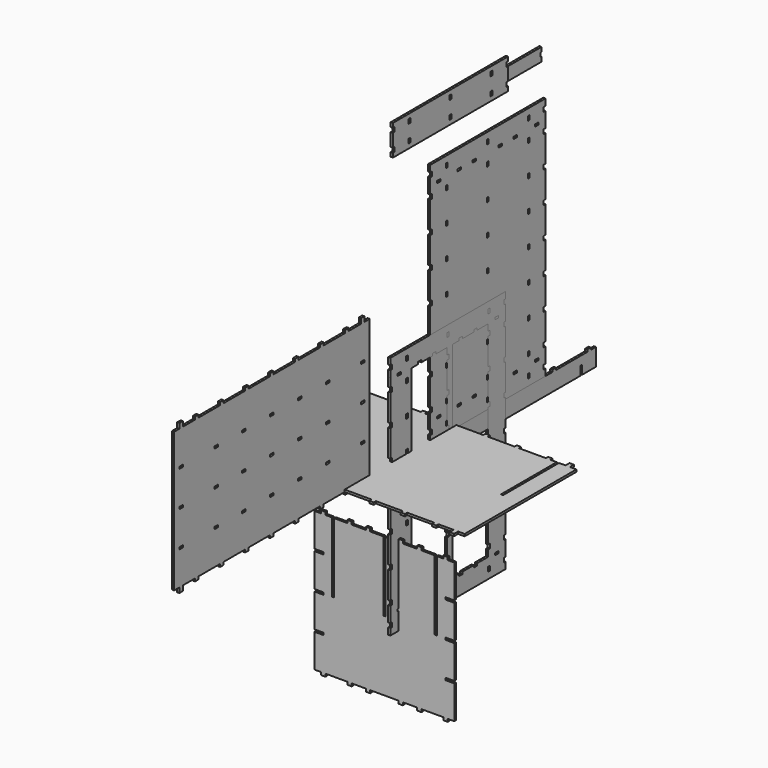
from build123d import *

# Parameters (mm, degrees)
F1_DEPTH  = 3.175
F3_DEPTH  = 3.175
F5_DEPTH  = 3.175
F6_W      = 6.35
F6_H      = 3.175
F7_DEPTH  = 3.175
F8_W      = 6.35
F8_H      = 3.175
F8_W_2    = 3.175
F8_H_2    = 6.35
F9_DEPTH  = 3.175
F10_W     = 6.35
F10_H     = 3.175
F10_W_2   = 3.175
F10_H_2   = 6.35
F11_DEPTH = 3.175
F12_W     = 3.175
F12_H     = 6.35
F13_DEPTH = 3.175
F14_W     = 3.175
F14_H     = 6.35
F15_DEPTH = 3.175


# Not quite as in the source:
# - ends of sketch curves that miss each other by under 0.0002 mm in the source are joined


with BuildPart() as f1:
    # F0 (on Top) → F1 (new body)
    with BuildSketch(Plane.XY):
        Polygon((-168.275, 101.5999987721), (-177.8, 101.5999987721), (-177.8, -101.6), (-168.275, -101.5999989401), (-168.275, -105.5687489401), (-168.275, -108.8707489401), (-161.925, -108.8707489401), (-161.925, -105.5687489401), (-161.925, -101.5999989401), (-152.4, -101.5999989401), (-149.225, -101.5999989401), (-139.7, -101.5999989401), (-139.7, -105.5687489401), (-133.35, -105.5687489401), (-133.35, -101.6000026982), (-94.1916666667, -101.5999986028), (-94.1916666667, -105.5687477122), (-87.8416666667, -105.5687477122), (-87.8416666667, -101.5999977122), (-48.6833333333, -101.5999977122), (-48.6833333333, -105.5687477122), (-42.3333333333, -105.5687477122), (-42.3333333333, -101.5999977122), (-3.175, -101.5999977122), (-3.175, -105.5687489401), (3.175, -105.5687489401), (3.175, -101.5999989401), (42.3333333333, -101.5999989401), (42.3333333333, -105.5687494621), (48.6833333333, -105.5687494621), (48.6833333333, -101.5999990721), (87.8416666667, -101.5999990721), (87.8416666667, -105.5687490984), (94.1916666667, -105.5687490984), (94.1916666667, -101.5999987721), (133.35, -101.5999987721), (133.35, -105.5687487721), (139.7, -105.5687487721), (139.7, -101.5999987721), (149.225, -101.5999989401), (152.4, -101.5999977122), (161.925, -101.5999977122), (161.925, -105.5687477122), (161.925, -108.8707477122), (168.275, -108.8707477122), (168.275, -105.5687477122), (168.275, -101.5999977122), (177.8, -101.5999977122), (177.8, 101.6), (168.275, 101.6), (168.275, 105.56875), (168.275, 108.87075), (161.925, 108.87075), (161.925, 105.56875), (161.925, 101.6), (152.4, 101.6), (152.4, 0), (149.225, 0), (149.225, 101.6), (139.7, 101.6), (139.7, 105.56875), (133.35, 105.56875), (133.35, 101.6000037581), (94.1916666667, 101.5999996627), (94.1916666667, 105.5687487721), (87.8416666667, 105.5687487721), (87.8416666667, 101.5999987721), (48.6833333333, 101.5999987721), (48.6833333333, 105.5687487721), (42.3333333333, 105.5687487721), (42.3333333333, 101.5999987721), (3.175, 101.5999987721), (3.175, 105.56875), (-3.175, 105.56875), (-3.175, 101.6), (-42.3333333333, 101.6), (-42.3333333333, 105.568750522), (-48.6833333333, 105.568750522), (-48.6833333333, 101.600000132), (-87.8416666667, 101.600000132), (-87.8416666667, 105.5687501583), (-94.1916666667, 105.5687501583), (-94.1916666667, 101.5999998321), (-133.35, 101.5999998321), (-133.35, 105.5687498321), (-139.7, 105.5687498321), (-139.7, 101.5999998321), (-149.225, 101.6), (-149.225, 0), (-152.4, 0), (-152.4, 101.6), (-161.925, 101.5999987721), (-161.925, 105.5687487721), (-161.925, 108.8707487721), (-168.275, 108.8707487721), (-168.275, 105.5687487721), align=None)
    extrude(amount=F1_DEPTH)


with BuildPart() as f3:
    # F2 (on Front) → F3 (new body)
    with BuildSketch(Plane.XZ):
        Polygon((-93.8661349833, -205.6803156889), (-93.8661349833, -104.0803156889), (-103.3911349833, -104.0803156889), (-103.3911349833, -100.1115656889), (-109.7411349833, -100.1115656889), (-109.7411349833, -104.0803156889), (-119.2661324751, -104.0803029335), (-119.2661349833, -152.4990656889), (-106.566134983, -152.4990656889), (-106.566134983, -155.6740656889), (-119.266135106, -155.6740656889), (-119.2661374807, -204.0928156889), (-106.5661374807, -204.0928156889), (-106.5661374807, -207.2678156889), (-119.2661350678, -207.2678156889), (-119.2661350678, -255.6865656889), (-106.5661349833, -255.6865656889), (-106.5661349833, -258.8615656889), (-119.2661349833, -258.8615656889), (-119.2661349833, -307.2803156889), (-109.7411349833, -307.2803156889), (-109.7411349833, -311.2490656889), (-103.3911349833, -311.2490656889), (-103.3911349833, -307.2803156889), (-93.8661374807, -307.2803284443), (-90.6911332881, -307.2803020477), (-71.6411332881, -307.2803020477), (-71.6411332881, -311.2490520477), (-65.2911332881, -311.2490520477), (-65.2911332881, -307.2803020477), (-44.6536332816, -307.2803020477), (-44.6536332816, -311.2490520477), (-38.3036332816, -311.2490520477), (-38.3036332816, -307.2803020477), (-19.2536332816, -307.2803020477), (-16.0786324859, -307.2803020477), (2.9713675141, -307.2803020477), (2.9713675141, -311.2490520477), (9.3213675141, -311.2490520477), (9.3213675141, -307.2803020477), (29.9588675141, -307.2803020477), (29.9588675141, -311.2490520477), (36.3088675141, -311.2490520477), (36.3088675141, -307.2803020477), (55.3588675141, -307.2803020477), (58.5338675141, -307.2803020477), (68.0588675141, -307.2803020477), (68.0588675141, -311.2490520477), (74.4088675141, -311.2490520477), (74.4088675141, -307.2803020477), (83.9338650167, -307.2803148031), (83.9338650167, -258.8615648031), (71.2338650164, -258.8615648031), (71.2338675138, -256.6073194046), (71.2338650164, -255.6865648031), (83.9338651394, -255.6865648031), (83.9338675141, -207.2678148031), (71.2338675141, -207.2678148031), (71.2338675141, -204.0928148031), (83.9338651012, -204.0928148031), (83.9338651012, -155.6740648031), (71.2338650167, -155.6740648031), (71.2338650167, -152.4990648031), (83.9338650167, -152.4990648031), (83.9338650167, -104.0803148031), (74.4088650167, -104.0803148031), (74.4088650059, -100.1115648031), (68.0588650059, -100.1115648031), (68.0588650059, -104.0803148031), (58.5338675141, -104.0803020477), (58.5338650167, -205.6803156889), (55.3588650167, -205.6803156889), (55.3588650167, -104.0803156889), (36.3088658124, -104.0803156889), (36.3088658124, -100.1115656889), (29.9588658124, -100.1115656889), (29.9588658124, -104.0803156889), (9.3213658124, -104.0803156889), (9.3213658124, -100.1115656889), (2.9713658124, -100.1115656889), (2.9713658124, -104.0803156889), (-16.0786341876, -104.0803156889), (-16.0786349833, -205.6803156889), (-19.2536349833, -205.6803156889), (-19.2536349833, -104.0803156889), (-38.3036349833, -104.0803156889), (-38.3036349833, -100.1115656889), (-44.6536349833, -100.1115656889), (-44.6536349833, -104.0803156889), (-65.2911349833, -104.0803156889), (-65.2911349833, -100.1115656889), (-71.6411349833, -100.1115656889), (-71.6411349833, -104.0803156889), (-90.6911349833, -104.0803156889), (-90.6911349833, -205.6803156889), align=None)
    extrude(amount=F3_DEPTH)


with BuildPart() as f5:
    # F4 (on Right) → F5 (new body)
    with BuildSketch(Plane.YZ):
        Polygon((9.525, 0), (0, 0), (0, -25.4), (25.4, -25.4), (25.4, -12.4706057832), (28.575, -12.4706057832), (28.575, -25.4), (327.025, -25.399999693), (327.025, -12.4706054762), (330.2, -12.4706054762), (330.2, -25.399999693), (355.6, -25.4000000594), (355.6, 0), (346.075, 0), (346.075, 3.175), (339.725, 3.175), (339.725, 0), (282.575, 0), (282.575, 3.175), (276.225, 3.175), (276.225, 0), (231.775, 0), (231.775, 3.175), (225.425, 3.175), (225.425, 0), (180.975, 0), (180.975, 3.175), (174.625, 3.175), (174.625, 0), (130.175, 0), (130.175, 3.175), (123.825, 3.175), (123.825, 0), (79.375, 0), (79.375, 3.175), (73.025, 3.175), (73.025, 0), (15.875, 0), (15.875, 3.175), (9.525, 3.175), align=None)
    extrude(amount=F5_DEPTH)


with BuildPart() as f7:
    # F6 (on Right) → F7 (new body)
    with BuildSketch(Plane.YZ):
        Polygon((-402.0784507751, 203.1999987721), (-411.6034507751, 203.1999987721), (-411.6034507751, 0), (-402.0784507751, 1.0599e-06), (-402.0784507751, -3.9687489401), (-402.0784497261, -7.2707477122), (-395.7284497261, -7.2707477122), (-395.7284507751, -3.9687489401), (-395.7284507751, 1.0599e-06), (-386.2034507751, 1.0599e-06), (-383.0284507751, 1.0599e-06), (-373.5034507751, 1.0599e-06), (-373.5034507751, -3.9687489401), (-367.1534507751, -3.9687489401), (-367.1534507751, -2.6982e-06), (-327.9951174418, 1.3972e-06), (-327.9951174418, -3.9687477122), (-321.6451174418, -3.9687477122), (-321.6451174418, 2.2878e-06), (-282.4867841085, 2.2878e-06), (-282.4867841085, -3.9687477122), (-276.1367841085, -3.9687477122), (-276.1367841085, 2.2878e-06), (-236.9784507751, 2.2878e-06), (-236.9784507751, -3.9687489401), (-230.6284507751, -3.9687489401), (-230.6284507751, 1.0599e-06), (-191.4701174418, 1.0599e-06), (-191.4701174418, -3.9687494621), (-185.1201174418, -3.9687494621), (-185.1201174418, 9.279e-07), (-145.9617841085, 9.279e-07), (-145.9617841085, -3.9687490984), (-139.6117841085, -3.9687490984), (-139.6117841085, 1.2279e-06), (-100.4534507752, 1.2279e-06), (-100.4534507752, -3.9687487721), (-94.1034507752, -3.9687487721), (-94.1034507752, 1.2279e-06), (-84.5784507752, 1.0599e-06), (-81.4034507752, 2.2878e-06), (-71.8784507752, 2.2878e-06), (-71.8784507752, -3.9687477122), (-71.8784507752, -7.2707477122), (-65.5284507752, -7.2707477122), (-65.5284507752, -3.9687477122), (-65.5284507752, 2.2878e-06), (-56.0034507752, 2.2878e-06), (-56.0034507752, 203.1999999999), (-65.5284507752, 203.1999999999), (-65.5284507752, 207.1687499999), (-65.5284507752, 210.4602605104), (-71.8784507752, 210.4602605104), (-71.8784507752, 207.1687499999), (-71.8784507752, 203.1999999999), (-81.4034507752, 203.1999999999), (-84.5784507752, 203.1999999999), (-94.1034507752, 203.1999999999), (-94.1034507752, 207.16875), (-100.4534507752, 207.16875), (-100.4534507752, 203.200045394), (-139.6117841085, 203.2000412986), (-139.6117841085, 207.1687487721), (-145.9617841085, 207.1687487721), (-145.9617841085, 203.1999987721), (-185.1201174418, 203.1999987721), (-185.1201174418, 207.1687487721), (-191.4701174418, 207.1687487721), (-191.4701174418, 203.1999987721), (-230.6284507752, 203.1999987721), (-230.6284507752, 207.16875), (-236.9784507752, 207.16875), (-236.9784507752, 203.2), (-276.1367841085, 203.2), (-276.1367841085, 207.168750522), (-282.4867841085, 207.168750522), (-282.4867841085, 203.200000132), (-321.6451174418, 203.200000132), (-321.6451174418, 207.1687501583), (-327.9951174418, 207.1687501583), (-327.9951174418, 203.1999998321), (-367.1534507752, 203.1999998321), (-367.1534507752, 207.1687498321), (-373.5034507752, 207.1687498321), (-373.5034507752, 203.1999998321), (-383.0284507752, 203.2), (-386.2034507751, 203.1999987721), (-395.7284507751, 203.1999987721), (-395.7284507751, 207.1687487721), (-395.7284507751, 210.460267498), (-402.0784507751, 210.460267498), (-402.0784507751, 207.1687487721), align=None)
        with Locations((-398.9034507752, 50.0062499999)):
            Rectangle(F6_W, F6_H, mode=Mode.SUBTRACT)
        with Locations((-335.4034507752, 50.0062499999)):
            Rectangle(F6_W, F6_H, mode=Mode.SUBTRACT)
        with Locations((-284.6034507752, 50.0062499999)):
            Rectangle(F6_W, F6_H, mode=Mode.SUBTRACT)
        with Locations((-233.8034507752, 50.0062499999)):
            Rectangle(F6_W, F6_H, mode=Mode.SUBTRACT)
        with Locations((-183.0034507752, 50.006246829)):
            Rectangle(F6_W, F6_H, mode=Mode.SUBTRACT)
        with Locations((-132.2034507752, 50.006246829)):
            Rectangle(F6_W, F6_H, mode=Mode.SUBTRACT)
        with Locations((-68.7034507752, 50.0062499999)):
            Rectangle(F6_W, F6_H, mode=Mode.SUBTRACT)
        with Locations((-398.9034507752, 101.5999999999)):
            Rectangle(F6_W, F6_H, mode=Mode.SUBTRACT)
        with Locations((-335.4034507752, 101.5999999999)):
            Rectangle(F6_W, F6_H, mode=Mode.SUBTRACT)
        with Locations((-398.9034507752, 153.1937499999)):
            Rectangle(F6_W, F6_H, mode=Mode.SUBTRACT)
        with Locations((-335.4034507752, 153.1937499999)):
            Rectangle(F6_W, F6_H, mode=Mode.SUBTRACT)
        with Locations((-284.6034507752, 101.5999999999)):
            Rectangle(F6_W, F6_H, mode=Mode.SUBTRACT)
        with Locations((-233.8034507752, 101.5999999999)):
            Rectangle(F6_W, F6_H, mode=Mode.SUBTRACT)
        with Locations((-284.6034507752, 153.1937499999)):
            Rectangle(F6_W, F6_H, mode=Mode.SUBTRACT)
        with Locations((-233.8034507752, 153.1937499999)):
            Rectangle(F6_W, F6_H, mode=Mode.SUBTRACT)
        with Locations((-183.0034507752, 101.599996829)):
            Rectangle(F6_W, F6_H, mode=Mode.SUBTRACT)
        with Locations((-183.0034507752, 153.193746829)):
            Rectangle(F6_W, F6_H, mode=Mode.SUBTRACT)
        with Locations((-132.2034507752, 101.599996829)):
            Rectangle(F6_W, F6_H, mode=Mode.SUBTRACT)
        with Locations((-68.7034507752, 101.5999999999)):
            Rectangle(F6_W, F6_H, mode=Mode.SUBTRACT)
        with Locations((-132.2034507752, 153.193746829)):
            Rectangle(F6_W, F6_H, mode=Mode.SUBTRACT)
        with Locations((-68.7034507752, 153.1937499999)):
            Rectangle(F6_W, F6_H, mode=Mode.SUBTRACT)
    extrude(amount=F7_DEPTH)


with BuildPart() as f9:
    # F8 (on Right) → F9 (new body)
    with BuildSketch(Plane.YZ):
        Polygon((54.0407858789, 9.5250001177), (54.0407858789, 0), (263.5907858789, 0), (263.5907871068, 9.5249983788), (260.4157871068, 9.5249983788), (260.4157871068, 15.8749983788), (263.5907871068, 15.8749983788), (263.5907871068, 25.3999983788), (263.5907898064, 28.5749983788), (263.5907899743, 38.0999983788), (260.4157899743, 38.0999983788), (260.4157899743, 44.4499983788), (263.5907899743, 44.4499983788), (263.5907899743, 83.6083317121), (260.4157899743, 83.6083317121), (260.4157899743, 89.9583317121), (263.5907899743, 89.9583317121), (263.5907899743, 129.1166650454), (260.4157899743, 129.1166650454), (260.4157899743, 135.4666650454), (263.5907899743, 135.4666650454), (263.5907899743, 174.6249983788), (260.4157899743, 174.6249983788), (260.4157899743, 180.9749983788), (263.5907899743, 180.9749983788), (263.5907899743, 220.1333317121), (260.4157899743, 220.1333317121), (260.4157899743, 226.4833317121), (263.5907899743, 226.4833317121), (263.5907899743, 265.6416650454), (260.4157899743, 265.6416650454), (260.4157899743, 271.9916650454), (263.5907899743, 271.9916650454), (263.5907858789, 311.1499983788), (260.4157858789, 311.1499983788), (260.4157858789, 317.4999983788), (263.5907858789, 317.4999983788), (263.5907858789, 327.0249983788), (263.5907858789, 330.1999983788), (263.5907858789, 339.7249983788), (260.4157858789, 339.7249983788), (260.4157858789, 346.0749983788), (263.5907858789, 346.0749983788), (263.5907858789, 355.6), (54.0407858789, 355.6), (54.040784651, 346.0750001177), (57.215784651, 346.0750001177), (57.215784651, 339.7250001177), (54.040784651, 339.7250001177), (54.040784651, 330.2000001177), (54.0407819514, 327.0250001177), (54.0407817835, 317.5000001177), (57.2157817835, 317.5000001177), (57.2157817835, 311.1500001177), (54.0407817835, 311.1500001177), (54.0407817835, 271.9916667844), (57.2157817835, 271.9916667844), (57.2157817835, 265.6416667844), (54.0407817835, 265.6416667844), (54.0407817835, 226.4833334511), (57.2157817835, 226.4833334511), (57.2157817835, 220.1333334511), (54.0407817835, 220.1333334511), (54.0407817835, 180.9750001177), (57.2157817835, 180.9750001177), (57.2157817835, 174.6250001177), (54.0407817835, 174.6250001177), (54.0407817835, 135.4666667844), (57.2157817835, 135.4666667844), (57.2157817835, 129.1166667844), (54.0407817835, 129.1166667844), (54.0407817835, 89.9583334511), (57.2157817835, 89.9583334511), (57.2157817835, 83.6083334511), (54.0407817835, 83.6083334511), (54.0407858789, 44.4500001177), (57.2157858789, 44.4500001177), (57.2157858789, 38.1000001177), (54.0407858789, 38.1000001177), (54.0407858789, 28.5750001177), (54.0407858789, 25.4000001177), (54.0407858789, 15.8750001177), (57.2157858789, 15.8750001177), (57.2157858789, 9.5250001177), align=None)
        with Locations((69.9157858789, 26.9875)):
            Rectangle(F8_W, F8_H, mode=Mode.SUBTRACT)
        with Locations((84.2032858789, 12.7)):
            Rectangle(F8_W_2, F8_H_2, mode=Mode.SUBTRACT)
        with Locations((84.2032858789, 41.275)):
            Rectangle(F8_W_2, F8_H_2, mode=Mode.SUBTRACT)
        with Locations((84.2032817835, 86.7833333333)):
            Rectangle(F8_W_2, F8_H_2, mode=Mode.SUBTRACT)
        with Locations((107.2121954441, 26.9875)):
            Rectangle(F8_W, F8_H, mode=Mode.SUBTRACT)
        with Locations((134.1997033834, 26.9875)):
            Rectangle(F8_W, F8_H, mode=Mode.SUBTRACT)
        with Locations((158.8157830114, 86.7833317121)):
            Rectangle(F8_W_2, F8_H_2, mode=Mode.SUBTRACT)
        with Locations((84.2032817835, 132.2916666667)):
            Rectangle(F8_W_2, F8_H_2, mode=Mode.SUBTRACT)
        with Locations((158.8157830114, 132.2916650454)):
            Rectangle(F8_W_2, F8_H_2, mode=Mode.SUBTRACT)
        with Locations((158.8157830114, 177.7999983788)):
            Rectangle(F8_W_2, F8_H_2, mode=Mode.SUBTRACT)
        with Locations((158.8157871068, 12.6999983788)):
            Rectangle(F8_W_2, F8_H_2, mode=Mode.SUBTRACT)
        with Locations((158.8157871068, 41.2749983788)):
            Rectangle(F8_W_2, F8_H_2, mode=Mode.SUBTRACT)
        with Locations((181.8247041792, 26.9875)):
            Rectangle(F8_W, F8_H, mode=Mode.SUBTRACT)
        with Locations((208.8122041792, 26.9875)):
            Rectangle(F8_W, F8_H, mode=Mode.SUBTRACT)
        with Locations((233.4282871068, 12.6999983788)):
            Rectangle(F8_W_2, F8_H_2, mode=Mode.SUBTRACT)
        with Locations((233.4282871068, 41.2749983788)):
            Rectangle(F8_W_2, F8_H_2, mode=Mode.SUBTRACT)
        with Locations((247.7157858789, 26.9874962843)):
            Rectangle(F8_W, F8_H, mode=Mode.SUBTRACT)
        with Locations((233.4282830114, 86.7833317121)):
            Rectangle(F8_W_2, F8_H_2, mode=Mode.SUBTRACT)
        with Locations((233.4282830114, 132.2916650454)):
            Rectangle(F8_W_2, F8_H_2, mode=Mode.SUBTRACT)
        with Locations((233.4282830114, 177.7999983788)):
            Rectangle(F8_W_2, F8_H_2, mode=Mode.SUBTRACT)
        with Locations((84.2032817835, 177.8)):
            Rectangle(F8_W_2, F8_H_2, mode=Mode.SUBTRACT)
        with Locations((84.2032817835, 223.3083333333)):
            Rectangle(F8_W_2, F8_H_2, mode=Mode.SUBTRACT)
        with Locations((158.8157830114, 223.3083317121)):
            Rectangle(F8_W_2, F8_H_2, mode=Mode.SUBTRACT)
        with Locations((84.2032817835, 268.8166666667)):
            Rectangle(F8_W_2, F8_H_2, mode=Mode.SUBTRACT)
        with Locations((69.9157858789, 328.6125)):
            Rectangle(F8_W, F8_H, mode=Mode.SUBTRACT)
        with Locations((84.2032817835, 314.325)):
            Rectangle(F8_W_2, F8_H_2, mode=Mode.SUBTRACT)
        with Locations((84.203284651, 342.9)):
            Rectangle(F8_W_2, F8_H_2, mode=Mode.SUBTRACT)
        with Locations((158.8157830114, 268.8166650454)):
            Rectangle(F8_W_2, F8_H_2, mode=Mode.SUBTRACT)
        with Locations((107.2121954441, 328.6125)):
            Rectangle(F8_W, F8_H, mode=Mode.SUBTRACT)
        with Locations((134.1997033834, 328.6125)):
            Rectangle(F8_W, F8_H, mode=Mode.SUBTRACT)
        with Locations((158.8157830114, 314.3249983788)):
            Rectangle(F8_W_2, F8_H_2, mode=Mode.SUBTRACT)
        with Locations((158.8157858789, 342.8999983788)):
            Rectangle(F8_W_2, F8_H_2, mode=Mode.SUBTRACT)
        with Locations((233.4282830114, 223.3083317121)):
            Rectangle(F8_W_2, F8_H_2, mode=Mode.SUBTRACT)
        with Locations((181.8247041792, 328.6125)):
            Rectangle(F8_W, F8_H, mode=Mode.SUBTRACT)
        with Locations((208.8122041792, 328.6125)):
            Rectangle(F8_W, F8_H, mode=Mode.SUBTRACT)
        with Locations((233.4282830114, 268.8166650454)):
            Rectangle(F8_W_2, F8_H_2, mode=Mode.SUBTRACT)
        with Locations((233.4282830114, 314.3249983788)):
            Rectangle(F8_W_2, F8_H_2, mode=Mode.SUBTRACT)
        with Locations((233.4282858789, 342.8999983788)):
            Rectangle(F8_W_2, F8_H_2, mode=Mode.SUBTRACT)
        with Locations((247.7157858789, 328.6124962843)):
            Rectangle(F8_W, F8_H, mode=Mode.SUBTRACT)
    extrude(amount=F9_DEPTH)


with BuildPart() as f11:
    # F10 (on Right) → F11 (new body)
    with BuildSketch(Plane.YZ):
        Polygon((-18.3669430935, -208.1636050716), (-18.3669430935, -217.6886051893), (191.1830569065, -217.6886051893), (191.1830569065, -208.1636068106), (188.0080581344, -208.1636068106), (188.0080581344, -201.8136068106), (191.1830581344, -201.8136068106), (191.1830569065, -192.2886068106), (191.1830569065, -189.1136068106), (191.1830569065, -179.5886068106), (188.0080610019, -179.5886068106), (188.0080610019, -173.2386068106), (191.1830610019, -173.2386068106), (191.1830569065, -134.0802734772), (188.0080610019, -134.0802734772), (188.0080610019, -127.7302734772), (191.1830610019, -127.7302734772), (191.1830569065, -88.5719401439), (188.0080610019, -88.5719401439), (188.0080610019, -82.2219401439), (191.1830610019, -82.2219401439), (191.1830569065, -43.0636068106), (188.0080610019, -43.0636068106), (188.0080610019, -36.7136068106), (191.1830610019, -36.7136068106), (191.1830569065, 2.4447265228), (188.0080610019, 2.4447265228), (188.0080610019, 8.7947265228), (191.1830610019, 8.7947265228), (191.1830569065, 47.9530598561), (188.0080610019, 47.9530598561), (188.0080610019, 54.3030598561), (191.1830610019, 54.3030598561), (191.1830569065, 93.4613931894), (188.0080569065, 93.4613931894), (188.0080569065, 99.8113931894), (191.1830569065, 99.8113931894), (191.1830569065, 109.3363931894), (191.1830569065, 112.5113931894), (191.1830569065, 122.0363931894), (188.0080569065, 122.0363931894), (188.0080569065, 128.3863931894), (191.1830569065, 128.3863931894), (191.1830569065, 137.9113948107), (-18.3669430935, 137.9113948107), (-18.3669430935, 128.3863949284), (-15.1919443213, 128.3863949284), (-15.1919443213, 122.0363949284), (-18.3669443213, 122.0363949284), (-18.3669430935, 112.5113949284), (-18.3669430935, 109.3363949284), (-18.3669430935, 99.8113949284), (-15.1919471889, 99.8113949284), (-15.1919471889, 93.4613949284), (-18.3669471889, 93.4613949284), (-18.3669430935, 54.3030615951), (-15.1919471889, 54.3030615951), (-15.1919471889, 47.9530615951), (-18.3669471889, 47.9530615951), (-18.3669430935, 8.7947282617), (-15.1919471889, 8.7947282617), (-15.1919471889, 2.4447282617), (-18.3669471889, 2.4447282617), (-18.3669430935, -36.7136050716), (-15.1919471889, -36.7136050716), (-15.1919471889, -43.0636050716), (-18.3669471889, -43.0636050716), (-18.3669430935, -82.2219384049), (-15.1919471889, -82.2219384049), (-15.1919471889, -88.5719384049), (-18.3669471889, -88.5719384049), (-18.3669430935, -127.7302717383), (-15.1919471889, -127.7302717383), (-15.1919471889, -134.0802717383), (-18.3669471889, -134.0802717383), (-18.3669430935, -173.2386050716), (-15.1919430935, -173.2386050716), (-15.1919430935, -179.5886050716), (-18.3669430935, -179.5886050716), (-18.3669430935, -189.1136050716), (-18.3669430935, -192.2886050716), (-18.3669430935, -201.8136050716), (-15.1919430935, -201.8136050716), (-15.1919430935, -208.1636050716), align=None)
        with Locations((-2.4919430935, -190.7011051893)):
            Rectangle(F10_W, F10_H, mode=Mode.SUBTRACT)
        with Locations((11.7955569065, -204.9886051893)):
            Rectangle(F10_W_2, F10_H_2, mode=Mode.SUBTRACT)
        with Locations((11.7955569065, -176.4136051893)):
            Rectangle(F10_W_2, F10_H_2, mode=Mode.SUBTRACT)
        with Locations((11.7955528111, -130.905271856)):
            Rectangle(F10_W_2, F10_H_2, mode=Mode.SUBTRACT)
        with Locations((11.7955528111, -85.3969385227)):
            Rectangle(F10_W_2, F10_H_2, mode=Mode.SUBTRACT)
        with Locations((11.7955528111, -39.8886051893)):
            Rectangle(F10_W_2, F10_H_2, mode=Mode.SUBTRACT)
        with Locations((86.4080581344, -204.9886068106)):
            Rectangle(F10_W_2, F10_H_2, mode=Mode.SUBTRACT)
        with Locations((161.0205581344, -204.9886068106)):
            Rectangle(F10_W_2, F10_H_2, mode=Mode.SUBTRACT)
        with Locations((175.3080569065, -190.701108905)):
            Rectangle(F10_W, F10_H, mode=Mode.SUBTRACT)
        Polygon((139.5794752068, -192.2886051893), (133.2294752068, -192.2886051893), (133.2294752068, -189.1235006809), (112.5919752068, -189.1235006809), (112.5919752068, -192.2886051893), (106.2419752068, -192.2886051893), (106.2419752068, -189.1235006809), (94.3239471829, -189.1235006809), (94.3239471829, -189.1136051893), (94.3239471829, 102.976496172), (94.3239471829, 109.3264924526), (159.387571255, 109.3264924526), (159.387571255, 102.976496172), (159.387571255, 99.8014945507), (162.562571255, 99.8014945507), (162.562571255, 93.4514945507), (159.387571255, 93.4514945507), (159.387571255, 54.2931612174), (162.562571255, 54.2931612174), (162.562571255, 47.9431612174), (159.387571255, 47.9431612174), (159.387571255, 8.784827884), (162.562571255, 8.784827884), (162.562571255, 2.434827884), (159.387571255, 2.434827884), (159.387571255, -36.7235054493), (162.562571255, -36.7235054493), (162.562571255, -43.0735054493), (159.387571255, -43.0735054493), (159.387571255, -82.2318387826), (162.562571255, -82.2318387826), (162.562571255, -88.5818387826), (159.387571255, -88.5818387826), (159.387571255, -127.740172116), (162.562571255, -127.740172116), (162.562571255, -134.090172116), (159.387571255, -134.090172116), (159.387571255, -173.2485054493), (162.562571255, -173.2485054493), (162.562571255, -179.5985054493), (159.387571255, -179.5985054493), (159.387571255, -182.773503828), (159.387571255, -189.1235006809), (139.5794752068, -189.1235006809), align=None, mode=Mode.SUBTRACT)
        with Locations((11.7955528111, 5.619728144)):
            Rectangle(F10_W_2, F10_H_2, mode=Mode.SUBTRACT)
        Polygon((64.9669744111, -192.2886051893), (58.6169744111, -192.2886051893), (58.6169744111, -189.1136051893), (37.9794664717, -189.1136051893), (37.9794664717, -192.2886051893), (31.6294664717, -192.2886051893), (31.6294664717, -189.1136051893), (19.7330569065, -189.1136051893), (19.7330569065, 109.3363948107), (31.6294664717, 109.3363948107), (31.6294664717, 112.5113948107), (37.9794664717, 112.5113948107), (37.9794664717, 109.3363948107), (58.6169744111, 109.3363948107), (58.6169744111, 112.5113948107), (64.9669744111, 112.5113948107), (64.9669744111, 109.3363948107), (84.7989471829, 109.3363948107), (84.7989471829, 99.8014945507), (87.9739471829, 99.8014945507), (87.9739471829, 93.4514945507), (84.7989471829, 93.4514945507), (84.7989471829, 54.2931612174), (87.9739471829, 54.2931612174), (87.9739471829, 47.9431612174), (84.7989471829, 47.9431612174), (84.7989471829, 8.784827884), (87.9739471829, 8.784827884), (87.9739471829, 2.434827884), (84.7989471829, 2.434827884), (84.7989471829, -36.7235054493), (87.9739471829, -36.7235054493), (87.9739471829, -43.0735054493), (84.7989471829, -43.0735054493), (84.7989471829, -82.2318387826), (87.9739471829, -82.2318387826), (87.9739471829, -88.5818387826), (84.7989471829, -88.5818387826), (84.7989471829, -127.740172116), (87.9739471829, -127.740172116), (87.9739471829, -134.090172116), (84.7989471829, -134.090172116), (84.7989471829, -173.2485054493), (87.9739471829, -173.2485054493), (87.9739471829, -179.5985054493), (84.7989471829, -179.5985054493), (84.7989471829, -189.1136051893), (64.9669744111, -189.1136051893), align=None, mode=Mode.SUBTRACT)
        with Locations((11.7955528111, 51.1280614773)):
            Rectangle(F10_W_2, F10_H_2, mode=Mode.SUBTRACT)
        with Locations((-2.4919430935, 110.9238948107)):
            Rectangle(F10_W, F10_H, mode=Mode.SUBTRACT)
        with Locations((11.7955528111, 96.6363948107)):
            Rectangle(F10_W_2, F10_H_2, mode=Mode.SUBTRACT)
        with Locations((11.7955556787, 125.2113948114)):
            Rectangle(F10_W_2, F10_H_2, mode=Mode.SUBTRACT)
        with Locations((109.4169752068, 110.9238948107)):
            Rectangle(F10_W, F10_H, mode=Mode.SUBTRACT)
        with Locations((86.4080569065, 125.2113931962)):
            Rectangle(F10_W_2, F10_H_2, mode=Mode.SUBTRACT)
        with Locations((136.4044752068, 110.9238948107)):
            Rectangle(F10_W, F10_H, mode=Mode.SUBTRACT)
        with Locations((161.0205569065, 125.2113931894)):
            Rectangle(F10_W_2, F10_H_2, mode=Mode.SUBTRACT)
        with Locations((175.3080569065, 110.923891095)):
            Rectangle(F10_W, F10_H, mode=Mode.SUBTRACT)
    extrude(amount=F11_DEPTH)


with BuildPart() as f13:
    # F12 (on face) → F13 (new body)
    with BuildSketch(Plane.YZ.offset(3.175)):
        Polygon((191.8267451406, 433.2376080513), (191.8267451406, 439.5876080513), (-17.7232548594, 439.5876080513), (-17.7232548594, 433.2376097903), (-14.5482548594, 433.2376097903), (-14.5482548594, 426.8876097903), (-17.7232548594, 426.8876097903), (-17.7232548594, 407.8376080513), (-14.5482548594, 407.8376080513), (-14.5482548594, 401.4876080513), (-17.7232548594, 401.4876080513), (-17.7232548594, 395.1376080513), (191.8267451406, 395.1376080513), (191.8267451406, 401.4876063123), (188.6517451406, 401.4876063123), (188.6517451406, 407.8376063123), (191.8267451406, 407.8376063123), (191.8267451406, 426.8876080513), (188.6517451406, 426.8876080513), (188.6517451406, 433.2376080513), align=None)
        with Locations((12.4392451406, 404.6626079336)):
            Rectangle(F12_W, F12_H, mode=Mode.SUBTRACT)
        with Locations((87.0517463684, 404.6626063123)):
            Rectangle(F12_W, F12_H, mode=Mode.SUBTRACT)
        with Locations((161.6642463684, 404.6626063123)):
            Rectangle(F12_W, F12_H, mode=Mode.SUBTRACT)
        with Locations((12.4392451406, 430.0626096725)):
            Rectangle(F12_W, F12_H, mode=Mode.SUBTRACT)
        with Locations((87.0517463684, 430.0626080513)):
            Rectangle(F12_W, F12_H, mode=Mode.SUBTRACT)
        with Locations((161.6642463684, 430.0626080513)):
            Rectangle(F12_W, F12_H, mode=Mode.SUBTRACT)
    extrude(amount=F13_DEPTH)


with BuildPart() as f15:
    # F14 (on face) → F15 (new body)
    with BuildSketch(Plane(origin=(0, 0, 0), x_dir=(0, -1, 0), z_dir=(-1, 0, 0))):
        Polygon((-260.4157899743, 409.2008663177), (-260.4157899743, 402.8508663177), (-155.6407899743, 402.8508663177), (-155.6407899743, 409.2008663177), (-158.8157899743, 409.2008663177), (-158.8157899743, 415.5508663177), (-155.6407899743, 415.5508663177), (-155.6407899743, 421.9008663177), (-260.4157899743, 421.9008663177), (-260.4157899743, 415.5508663177), (-258.8282899743, 415.5508663177), (-258.8282899743, 409.2008663177), align=None)
        with Locations((-185.8032899743, 412.3758663177)):
            Rectangle(F14_W, F14_H, mode=Mode.SUBTRACT)
        Polygon((-155.6407899743, 409.2008663177), (-155.6407899743, 402.8508663177), (-50.8657899743, 402.8508663177), (-50.8657899743, 409.2008663177), (-52.4532899743, 409.2008663177), (-52.4532899743, 415.5508663177), (-50.8657899743, 415.5508663177), (-50.8657899743, 421.9008663177), (-155.6407899743, 421.9008663177), (-155.6407899743, 415.5508663177), (-152.4657899743, 415.5508663177), (-152.4657899743, 409.2008663177), align=None)
        with Locations((-125.4782899743, 412.3758663177)):
            Rectangle(F14_W, F14_H, mode=Mode.SUBTRACT)
    extrude(amount=F15_DEPTH)


solid = Compound([f1.part, f3.part, f5.part, f7.part, f9.part, f11.part, f13.part, f15.part])
